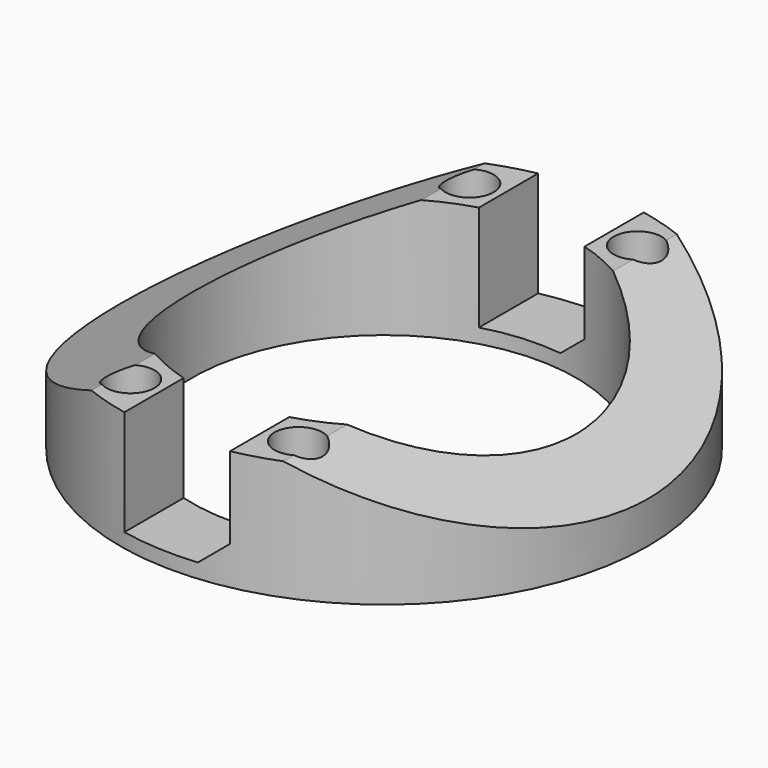
from build123d import *

# Parameters (mm, degrees)
F0_R             = 55
F1_DEPTH         = 25
F3_DEPTH         = 55.001
F3_DEPTH_BACK    = 55.001
F5_DEPTH         = 55.001
F5_DEPTH_BACK    = 55.001
F6_R             = 5
F8_DEPTH         = 20
F8_COPIES2_COUNT = 2


# Not quite as in the source:
# - a pattern or mirror of a feature is missing from the dataset's text; its kind, count and spacing are read off the source's solid


with BuildPart() as f1:
    # F0 (on Top) → F1 (new body)
    with BuildSketch(Plane.XY):
        Circle(F0_R)
        with BuildLine():
            ThreePointArc((39.9217985567, -2.5), (-40, 0), (39.9217985567, 2.5))
            ThreePointArc((39.9217985567, 2.5), (40, 0), (39.9217985567, -2.5))
        make_face(mode=Mode.SUBTRACT)
    extrude(amount=F1_DEPTH)

    # F2 (on Front) → F3 (cut, two sides)
    with BuildSketch(Plane.XZ) as f3_sk:
        Polygon((62.8901384102, 25), (20, 25), (62.8901384102, 5), align=None)
        Polygon((-62.8901384102, 5), (-20, 25), (-62.8901384102, 25), align=None)
    extrude(amount=-F3_DEPTH, mode=Mode.SUBTRACT)
    extrude(f3_sk.sketch, amount=F3_DEPTH_BACK, mode=Mode.SUBTRACT)

    # F4 (on Front) → F5 (cut, two sides)
    with BuildSketch(Plane.XZ) as f5_sk:
        Polygon((11, 25), (-11, 25), (-11, 3), (5, 3), (11, 8), align=None)
    extrude(amount=F5_DEPTH, mode=Mode.SUBTRACT)
    extrude(f5_sk.sketch, amount=-F5_DEPTH_BACK, mode=Mode.SUBTRACT)

    # F6 (on face) → F8 (cut, through all)
    with BuildSketch(Plane.XY.offset(25)):
        with Locations((17.5, 44.1549887905)):
            Circle(F6_R)
    f8 = extrude(amount=-F8_DEPTH, mode=Mode.SUBTRACT)

    # F8_copies: F8 across plane
    add(f8.mirror(Plane(origin=(0, 0, 0), x_dir=(0, 0, -1), z_dir=(-1, 0, 0))), mode=Mode.SUBTRACT)

    # F8_copies1: F8 across plane
    add(f8.mirror(Plane(origin=(0, 0, 0), x_dir=(0, 0, -1), z_dir=(0, -1, 0))), mode=Mode.SUBTRACT)

    # F8_copies2: F8 ×2 about axis
    f8_copies2_axis = Axis((0, 0, 0), (0, 0, 1))
    for i in range(1, F8_COPIES2_COUNT):
        add(f8.rotate(f8_copies2_axis, i * 360 / F8_COPIES2_COUNT), mode=Mode.SUBTRACT)


solid = f1.part
